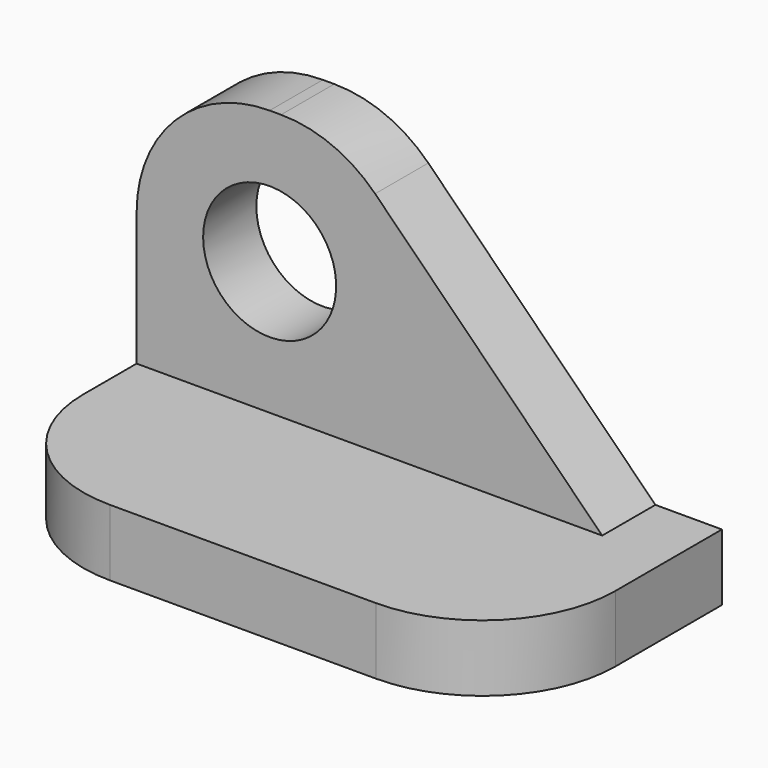
from build123d import *

# Parameters (mm, degrees)
F0_W     = 203.2
F0_H     = 101.6
F1_DEPTH = 25.4
F2_R     = 50.8
F3_W     = 177.8
F3_H     = 25.4
F4_DEPTH = 25.4
F5_DEPTH = 101.6
F6_SIZE2 = 101.59999
F6_SIZE  = 101.59999
F7_R     = 50.8
F9_D     = 50.8


# Not quite as in the source:
# - a fillet or chamfer is up to 0.001 mm smaller than in the source, because OpenCascade refuses the exact size


with BuildPart() as f1:
    # F0 (on Top) → F1 (new body)
    with BuildSketch(Plane.XY):
        with Locations((52.4225905538, -10.3211964953)):
            Rectangle(F0_W, F0_H)
    extrude(amount=F1_DEPTH)

    # F2
    f2_edges = [f1.edges().sort_by_distance(p)[0] for p in [
        (-49.177409, -61.121196, 12.7),
        (154.022591, -61.121196, 12.7),
    ]]
    fillet(f2_edges, radius=F2_R)

    # F3 (on face) → F4 (join)
    with BuildSketch(Plane.XY.offset(25.4)):
        with Locations((39.7225905538, 27.7788035047)):
            Rectangle(F3_W, F3_H)
    extrude(amount=F4_DEPTH)

    # F3 (on face) → F5 (join)
    with BuildSketch(Plane.XY.offset(25.4)):
        with Locations((39.7225905538, 27.7788035047)):
            Rectangle(F3_W, F3_H)
    extrude(amount=F5_DEPTH)

    # F6 (size 101.6 and 101.6 in the source; OpenCascade refuses exactly that, so slightly less here)
    f6_edges = [f1.edges().sort_by_distance(p)[0] for p in [
        (128.622591, 27.778804, 127),
    ]]
    chamfer(f6_edges, length=F6_SIZE, length2=F6_SIZE2)

    # F7
    f7_edges = [f1.edges().sort_by_distance(p)[0] for p in [
        (-49.177409, 27.778804, 127),
        (27.022601, 27.778804, 127),
    ]]
    fillet(f7_edges, radius=F7_R)

    # F9 (through all)
    with Locations(Plane.XZ.offset(-15.0788035047)):
        with Locations((1.6225905538, 76.2)):
            Hole(F9_D / 2)


solid = f1.part
